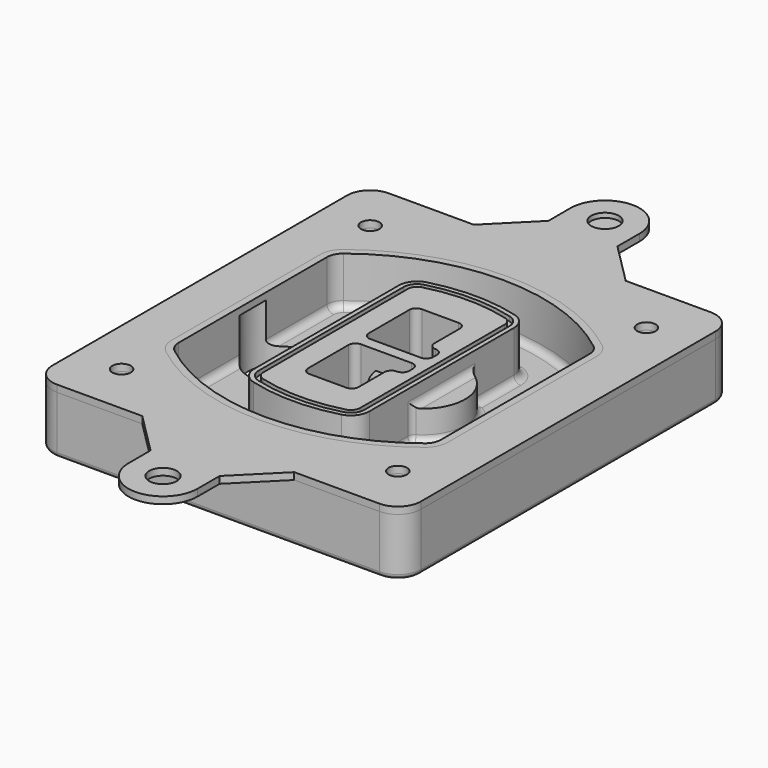
from build123d import *

# Parameters (mm, degrees)
F0_R      = 4
F1_DEPTH  = 25
F2_DEPTH  = 3
F3_DEPTH  = 18
F5_DEPTH  = 21
F6_DEPTH  = 2
F8_DEPTH  = 20
F9_DEPTH  = 16
F10_DEPTH = 25
F7_R      = 6
F7_R_2    = 4
F11_DEPTH = 6
F13_DEPTH = 9
F14_R     = 3
F15_R     = 2
F16_R     = 6
F16_R_2   = 4
F17_DEPTH = 3
F18_DEPTH = 1


# Not quite as in the source:
# - the program builds the solid bodies; features that only make, move or delete a surface that nothing else refers to are left out


with BuildPart() as f1:
    # F0 (on Top) → F1 (new body)
    with BuildSketch(Plane.XY):
        with BuildLine():
            ThreePointArc((-80, -80), (-77.0710678119, -87.0710678119), (-70, -90))
            Line((-70, -90), (70, -90))
            ThreePointArc((70, -90), (77.0710678119, -87.0710678119), (80, -80))
            Line((80, -80), (80, 80))
            ThreePointArc((80, 80), (77.0710678119, 87.0710678119), (70, 90))
            Line((70, 90), (-70, 90))
            ThreePointArc((-70, 90), (-77.0710678119, 87.0710678119), (-80, 80))
            Line((-80, 80), (-80, -80))
        make_face()
        with Locations((-60, -67.5)):
            Circle(F0_R, mode=Mode.SUBTRACT)
        with Locations((60, -67.5)):
            Circle(F0_R, mode=Mode.SUBTRACT)
        with Locations((-60, 67.5)):
            Circle(F0_R, mode=Mode.SUBTRACT)
        with BuildLine():
            ThreePointArc((-64, 40.2934422872), (-62.5820384798, 46.4328484224), (-58.6153846154, 51.3286200352))
            ThreePointArc((-58.6153846154, 51.3286200352), (0, 71.5), (58.6153846154, 51.3286200352))
            ThreePointArc((58.6153846154, 51.3286200352), (62.5820384798, 46.4328484224), (64, 40.2934422872))
            Line((64, 40.2934422872), (64, -40.2934422872))
            ThreePointArc((64, -40.2934422872), (62.5820384798, -46.4328484224), (58.6153846154, -51.3286200352))
            ThreePointArc((58.6153846154, -51.3286200352), (0, -71.5), (-58.6153846154, -51.3286200352))
            ThreePointArc((-58.6153846154, -51.3286200352), (-62.5820384798, -46.4328484224), (-64, -40.2934422872))
            Line((-64, -40.2934422872), (-64, 40.2934422872))
        make_face(mode=Mode.SUBTRACT)
        with Locations((60, 67.5)):
            Circle(F0_R, mode=Mode.SUBTRACT)
        with BuildLine():
            ThreePointArc((58.6153846154, 51.3286200352), (0, 71.5), (-58.6153846154, 51.3286200352))
            ThreePointArc((-58.6153846154, 51.3286200352), (-62.5820384798, 46.4328484224), (-64, 40.2934422872))
            Line((-64, 40.2934422872), (-64, -40.2934422872))
            ThreePointArc((-64, -40.2934422872), (-62.5820384798, -46.4328484224), (-58.6153846154, -51.3286200352))
            ThreePointArc((-58.6153846154, -51.3286200352), (0, -71.5), (58.6153846154, -51.3286200352))
            ThreePointArc((58.6153846154, -51.3286200352), (62.5820384798, -46.4328484224), (64, -40.2934422872))
            Line((64, -40.2934422872), (64, 40.2934422872))
            ThreePointArc((64, 40.2934422872), (62.5820384798, 46.4328484224), (58.6153846154, 51.3286200352))
        make_face()
        with BuildLine():
            Line((-60, -40.2934422872), (-60, 40.2934422872))
            ThreePointArc((-60, 40.2934422872), (-58.9871703427, 44.6787323838), (-56.1538461538, 48.1757121072))
            ThreePointArc((-56.1538461538, 48.1757121072), (0, 67.5), (56.1538461538, 48.1757121072))
            ThreePointArc((56.1538461538, 48.1757121072), (58.9871703427, 44.6787323838), (60, 40.2934422872))
            Line((60, 40.2934422872), (60, -40.2934422872))
            ThreePointArc((60, -40.2934422872), (58.9871703427, -44.6787323838), (56.1538461538, -48.1757121072))
            ThreePointArc((56.1538461538, -48.1757121072), (0, -67.5), (-56.1538461538, -48.1757121072))
            ThreePointArc((-56.1538461538, -48.1757121072), (-58.9871703427, -44.6787323838), (-60, -40.2934422872))
        make_face(mode=Mode.SUBTRACT)
        with BuildLine():
            ThreePointArc((-56.1538461538, 48.1757121072), (-58.9871703427, 44.6787323838), (-60, 40.2934422872))
            Line((-60, 40.2934422872), (-60, -40.2934422872))
            ThreePointArc((-60, -40.2934422872), (-58.9871703427, -44.6787323838), (-56.1538461538, -48.1757121072))
            ThreePointArc((-56.1538461538, -48.1757121072), (0, -67.5), (56.1538461538, -48.1757121072))
            ThreePointArc((56.1538461538, -48.1757121072), (58.9871703427, -44.6787323838), (60, -40.2934422872))
            Line((60, -40.2934422872), (60, 40.2934422872))
            ThreePointArc((60, 40.2934422872), (58.9871703427, 44.6787323838), (56.1538461538, 48.1757121072))
            ThreePointArc((56.1538461538, 48.1757121072), (0, 67.5), (-56.1538461538, 48.1757121072))
        make_face()
        with BuildLine():
            ThreePointArc((54.3076923077, 45.8110311612), (56.2910192399, 43.3631453548), (57, 40.2934422872))
            Line((57, 40.2934422872), (57, -40.2934422872))
            ThreePointArc((57, -40.2934422872), (56.2910192399, -43.3631453548), (54.3076923077, -45.8110311612))
            ThreePointArc((54.3076923077, -45.8110311612), (0, -64.5), (-54.3076923077, -45.8110311612))
            ThreePointArc((-54.3076923077, -45.8110311612), (-56.2910192399, -43.3631453548), (-57, -40.2934422872))
            Line((-57, -40.2934422872), (-57, 40.2934422872))
            ThreePointArc((-57, 40.2934422872), (-56.2910192399, 43.3631453548), (-54.3076923077, 45.8110311612))
            ThreePointArc((-54.3076923077, 45.8110311612), (0, 64.5), (54.3076923077, 45.8110311612))
        make_face(mode=Mode.SUBTRACT)
        with BuildLine():
            Line((57, -40.2934422872), (57, 40.2934422872))
            ThreePointArc((57, 40.2934422872), (56.2910192399, 43.3631453548), (54.3076923077, 45.8110311612))
            ThreePointArc((54.3076923077, 45.8110311612), (0, 64.5), (-54.3076923077, 45.8110311612))
            ThreePointArc((-54.3076923077, 45.8110311612), (-56.2910192399, 43.3631453548), (-57, 40.2934422872))
            Line((-57, 40.2934422872), (-57, -40.2934422872))
            ThreePointArc((-57, -40.2934422872), (-56.2910192399, -43.3631453548), (-54.3076923077, -45.8110311612))
            ThreePointArc((-54.3076923077, -45.8110311612), (0, -64.5), (54.3076923077, -45.8110311612))
            ThreePointArc((54.3076923077, -45.8110311612), (56.2910192399, -43.3631453548), (57, -40.2934422872))
        make_face()
    extrude(amount=-F1_DEPTH)

    # F0 (on Top) → F2 (join)
    with BuildSketch(Plane.XY):
        with BuildLine():
            ThreePointArc((-56.1538461538, 48.1757121072), (-58.9871703427, 44.6787323838), (-60, 40.2934422872))
            Line((-60, 40.2934422872), (-60, -40.2934422872))
            ThreePointArc((-60, -40.2934422872), (-58.9871703427, -44.6787323838), (-56.1538461538, -48.1757121072))
            ThreePointArc((-56.1538461538, -48.1757121072), (0, -67.5), (56.1538461538, -48.1757121072))
            ThreePointArc((56.1538461538, -48.1757121072), (58.9871703427, -44.6787323838), (60, -40.2934422872))
            Line((60, -40.2934422872), (60, 40.2934422872))
            ThreePointArc((60, 40.2934422872), (58.9871703427, 44.6787323838), (56.1538461538, 48.1757121072))
            ThreePointArc((56.1538461538, 48.1757121072), (0, 67.5), (-56.1538461538, 48.1757121072))
        make_face()
        with BuildLine():
            ThreePointArc((54.3076923077, 45.8110311612), (56.2910192399, 43.3631453548), (57, 40.2934422872))
            Line((57, 40.2934422872), (57, -40.2934422872))
            ThreePointArc((57, -40.2934422872), (56.2910192399, -43.3631453548), (54.3076923077, -45.8110311612))
            ThreePointArc((54.3076923077, -45.8110311612), (0, -64.5), (-54.3076923077, -45.8110311612))
            ThreePointArc((-54.3076923077, -45.8110311612), (-56.2910192399, -43.3631453548), (-57, -40.2934422872))
            Line((-57, -40.2934422872), (-57, 40.2934422872))
            ThreePointArc((-57, 40.2934422872), (-56.2910192399, 43.3631453548), (-54.3076923077, 45.8110311612))
            ThreePointArc((-54.3076923077, 45.8110311612), (0, 64.5), (54.3076923077, 45.8110311612))
        make_face(mode=Mode.SUBTRACT)
    extrude(amount=F2_DEPTH)

    # F0 (on Top) → F3 (cut)
    with BuildSketch(Plane.XY):
        with BuildLine():
            Line((57, -40.2934422872), (57, 40.2934422872))
            ThreePointArc((57, 40.2934422872), (56.2910192399, 43.3631453548), (54.3076923077, 45.8110311612))
            ThreePointArc((54.3076923077, 45.8110311612), (0, 64.5), (-54.3076923077, 45.8110311612))
            ThreePointArc((-54.3076923077, 45.8110311612), (-56.2910192399, 43.3631453548), (-57, 40.2934422872))
            Line((-57, 40.2934422872), (-57, -40.2934422872))
            ThreePointArc((-57, -40.2934422872), (-56.2910192399, -43.3631453548), (-54.3076923077, -45.8110311612))
            ThreePointArc((-54.3076923077, -45.8110311612), (0, -64.5), (54.3076923077, -45.8110311612))
            ThreePointArc((54.3076923077, -45.8110311612), (56.2910192399, -43.3631453548), (57, -40.2934422872))
        make_face()
    extrude(amount=-F3_DEPTH, mode=Mode.SUBTRACT)

    # F4 (on face) → F5 (join, through all)
    with BuildSketch(Plane.XY.offset(3)):
        with BuildLine():
            ThreePointArc((-25, -39.2465276821), (-23.3511545998, -44.1109737193), (-19.0842911877, -46.9702398883))
            ThreePointArc((-19.0842911877, -46.9702398883), (0, -49.5), (19.0842911877, -46.9702398883))
            ThreePointArc((19.0842911877, -46.9702398883), (23.3511545998, -44.1109737193), (25, -39.2465276821))
            Line((25, -39.2465276821), (25, 39.2465276821))
            ThreePointArc((25, 39.2465276821), (23.3511545998, 44.1109737193), (19.0842911877, 46.9702398883))
            ThreePointArc((19.0842911877, 46.9702398883), (0, 49.5), (-19.0842911877, 46.9702398883))
            ThreePointArc((-19.0842911877, 46.9702398883), (-23.3511545998, 44.1109737193), (-25, 39.2465276821))
            Line((-25, 39.2465276821), (-25, -39.2465276821))
        make_face()
        with BuildLine():
            ThreePointArc((18.5632183908, 45.0393118368), (21.7633659499, 42.89486221), (23, 39.2465276821))
            Line((23, 39.2465276821), (23, -39.2465276821))
            ThreePointArc((23, -39.2465276821), (21.7633659499, -42.89486221), (18.5632183908, -45.0393118368))
            ThreePointArc((18.5632183908, -45.0393118368), (0, -47.5), (-18.5632183908, -45.0393118368))
            ThreePointArc((-18.5632183908, -45.0393118368), (-21.7633659499, -42.89486221), (-23, -39.2465276821))
            Line((-23, -39.2465276821), (-23, 39.2465276821))
            ThreePointArc((-23, 39.2465276821), (-21.7633659499, 42.89486221), (-18.5632183908, 45.0393118368))
            ThreePointArc((-18.5632183908, 45.0393118368), (0, 47.5), (18.5632183908, 45.0393118368))
        make_face(mode=Mode.SUBTRACT)
        with BuildLine():
            Line((23, -39.2465276821), (23, 39.2465276821))
            ThreePointArc((23, 39.2465276821), (21.7633659499, 42.89486221), (18.5632183908, 45.0393118368))
            ThreePointArc((18.5632183908, 45.0393118368), (0, 47.5), (-18.5632183908, 45.0393118368))
            ThreePointArc((-18.5632183908, 45.0393118368), (-21.7633659499, 42.89486221), (-23, 39.2465276821))
            Line((-23, 39.2465276821), (-23, -39.2465276821))
            ThreePointArc((-23, -39.2465276821), (-21.7633659499, -42.89486221), (-18.5632183908, -45.0393118368))
            ThreePointArc((-18.5632183908, -45.0393118368), (0, -47.5), (18.5632183908, -45.0393118368))
            ThreePointArc((18.5632183908, -45.0393118368), (21.7633659499, -42.89486221), (23, -39.2465276821))
        make_face()
        with BuildLine():
            ThreePointArc((18.0421455939, 43.1083837852), (20.1755772999, 41.6787507007), (21, 39.2465276821))
            Line((21, 39.2465276821), (21, -39.2465276821))
            ThreePointArc((21, -39.2465276821), (20.1755772999, -41.6787507007), (18.0421455939, -43.1083837852))
            ThreePointArc((18.0421455939, -43.1083837852), (0, -45.5), (-18.0421455939, -43.1083837852))
            ThreePointArc((-18.0421455939, -43.1083837852), (-20.1755772999, -41.6787507007), (-21, -39.2465276821))
            Line((-21, -39.2465276821), (-21, 39.2465276821))
            ThreePointArc((-21, 39.2465276821), (-20.1755772999, 41.6787507007), (-18.0421455939, 43.1083837852))
            ThreePointArc((-18.0421455939, 43.1083837852), (0, 45.5), (18.0421455939, 43.1083837852))
        make_face(mode=Mode.SUBTRACT)
        with BuildLine():
            Line((21, -39.2465276821), (21, 39.2465276821))
            ThreePointArc((21, 39.2465276821), (20.1755772999, 41.6787507007), (18.0421455939, 43.1083837852))
            ThreePointArc((18.0421455939, 43.1083837852), (0, 45.5), (-18.0421455939, 43.1083837852))
            ThreePointArc((-18.0421455939, 43.1083837852), (-20.1755772999, 41.6787507007), (-21, 39.2465276821))
            Line((-21, 39.2465276821), (-21, -39.2465276821))
            ThreePointArc((-21, -39.2465276821), (-20.1755772999, -41.6787507007), (-18.0421455939, -43.1083837852))
            ThreePointArc((-18.0421455939, -43.1083837852), (0, -45.5), (18.0421455939, -43.1083837852))
            ThreePointArc((18.0421455939, -43.1083837852), (20.1755772999, -41.6787507007), (21, -39.2465276821))
        make_face()
        with BuildLine():
            Line((-8, -2.5), (14, -2.5))
            ThreePointArc((14, -2.5), (16.1213203436, -3.3786796564), (17, -5.5))
            Line((17, -5.5), (17, -7.5))
            ThreePointArc((17, -7.5), (16.1213203436, -9.6213203436), (14, -10.5))
            ThreePointArc((14, -10.5), (11.8786796564, -11.3786796564), (11, -13.5))
            Line((11, -13.5), (11, -27.5))
            ThreePointArc((11, -27.5), (10.1213203436, -29.6213203436), (8, -30.5))
            Line((8, -30.5), (-8, -30.5))
            ThreePointArc((-8, -30.5), (-10.1213203436, -29.6213203436), (-11, -27.5))
            Line((-11, -27.5), (-11, -5.5))
            ThreePointArc((-11, -5.5), (-10.1213203436, -3.3786796564), (-8, -2.5))
        make_face(mode=Mode.SUBTRACT)
        with BuildLine():
            ThreePointArc((-8, 2.5), (-10.1213203436, 3.3786796564), (-11, 5.5))
            Line((-11, 5.5), (-11, 27.5))
            ThreePointArc((-11, 27.5), (-10.1213203436, 29.6213203436), (-8, 30.5))
            Line((-8, 30.5), (8, 30.5))
            ThreePointArc((8, 30.5), (10.1213203436, 29.6213203436), (11, 27.5))
            Line((11, 27.5), (11, 13.5))
            ThreePointArc((11, 13.5), (11.8786796564, 11.3786796564), (14, 10.5))
            ThreePointArc((14, 10.5), (16.1213203436, 9.6213203436), (17, 7.5))
            Line((17, 7.5), (17, 5.5))
            ThreePointArc((17, 5.5), (16.1213203436, 3.3786796564), (14, 2.5))
            Line((14, 2.5), (-8, 2.5))
        make_face(mode=Mode.SUBTRACT)
    extrude(amount=-F5_DEPTH)

    # F4 (on face) → F6 (cut)
    with BuildSketch(Plane.XY.offset(3)):
        with BuildLine():
            Line((23, -39.2465276821), (23, 39.2465276821))
            ThreePointArc((23, 39.2465276821), (21.7633659499, 42.89486221), (18.5632183908, 45.0393118368))
            ThreePointArc((18.5632183908, 45.0393118368), (0, 47.5), (-18.5632183908, 45.0393118368))
            ThreePointArc((-18.5632183908, 45.0393118368), (-21.7633659499, 42.89486221), (-23, 39.2465276821))
            Line((-23, 39.2465276821), (-23, -39.2465276821))
            ThreePointArc((-23, -39.2465276821), (-21.7633659499, -42.89486221), (-18.5632183908, -45.0393118368))
            ThreePointArc((-18.5632183908, -45.0393118368), (0, -47.5), (18.5632183908, -45.0393118368))
            ThreePointArc((18.5632183908, -45.0393118368), (21.7633659499, -42.89486221), (23, -39.2465276821))
        make_face()
        with BuildLine():
            ThreePointArc((18.0421455939, 43.1083837852), (20.1755772999, 41.6787507007), (21, 39.2465276821))
            Line((21, 39.2465276821), (21, -39.2465276821))
            ThreePointArc((21, -39.2465276821), (20.1755772999, -41.6787507007), (18.0421455939, -43.1083837852))
            ThreePointArc((18.0421455939, -43.1083837852), (0, -45.5), (-18.0421455939, -43.1083837852))
            ThreePointArc((-18.0421455939, -43.1083837852), (-20.1755772999, -41.6787507007), (-21, -39.2465276821))
            Line((-21, -39.2465276821), (-21, 39.2465276821))
            ThreePointArc((-21, 39.2465276821), (-20.1755772999, 41.6787507007), (-18.0421455939, 43.1083837852))
            ThreePointArc((-18.0421455939, 43.1083837852), (0, 45.5), (18.0421455939, 43.1083837852))
        make_face(mode=Mode.SUBTRACT)
    extrude(amount=-F6_DEPTH, mode=Mode.SUBTRACT)

    # F7 (on face) → F8 (join)
    with BuildSketch(Plane(origin=(0, 0, -25), x_dir=(1, 0, 0), z_dir=(0, 0, -1))):
        with BuildLine():
            ThreePointArc((3.28842436, 0), (16.7567035675, 13.4682792075), (30.224982775, 0))
            Line((30.224982775, 0), (35.224982775, 0))
            ThreePointArc((35.224982775, 0), (16.7567035675, 18.4682792075), (-1.71157564, 0))
            Line((-1.71157564, 0), (3.28842436, 0))
        make_face()
        with BuildLine():
            Line((3.28842436, 0), (30.224982775, 0))
            ThreePointArc((30.224982775, 0), (16.7567035675, 13.4682792075), (3.28842436, 0))
        make_face()
        with BuildLine():
            ThreePointArc((3.28842436, 0), (16.7567035675, -13.4682792075), (30.224982775, 0))
            Line((30.224982775, 0), (3.28842436, 0))
        make_face()
        with BuildLine():
            Line((35.224982775, 0), (30.224982775, 0))
            ThreePointArc((30.224982775, 0), (16.7567035675, -13.4682792075), (3.28842436, 0))
            Line((3.28842436, 0), (-1.71157564, 0))
            ThreePointArc((-1.71157564, 0), (16.7567035675, -18.4682792075), (35.224982775, 0))
        make_face()
    extrude(amount=-F8_DEPTH)

    # F7 (on face) → F9 (cut)
    with BuildSketch(Plane(origin=(0, 0, -25), x_dir=(1, 0, 0), z_dir=(0, 0, -1))):
        with BuildLine():
            Line((3.28842436, 0), (30.224982775, 0))
            ThreePointArc((30.224982775, 0), (16.7567035675, 13.4682792075), (3.28842436, 0))
        make_face()
        with BuildLine():
            ThreePointArc((3.28842436, 0), (16.7567035675, -13.4682792075), (30.224982775, 0))
            Line((30.224982775, 0), (3.28842436, 0))
        make_face()
    extrude(amount=-F9_DEPTH, mode=Mode.SUBTRACT)

    # F7 (on face) → F10 (cut)
    with BuildSketch(Plane(origin=(0, 0, -25), x_dir=(1, 0, 0), z_dir=(0, 0, -1))):
        with BuildLine():
            Line((-59.0318229325, 0), (-32.0952645175, 0))
            ThreePointArc((-32.0952645175, 0), (-45.563543725, 13.4682792075), (-59.0318229325, 0))
        make_face()
        with BuildLine():
            ThreePointArc((-59.0318229325, 0), (-45.563543725, -13.4682792075), (-32.0952645175, 0))
            Line((-32.0952645175, 0), (-59.0318229325, 0))
        make_face()
    extrude(amount=-F10_DEPTH, mode=Mode.SUBTRACT)

    # F7 (on face) → F11 (cut)
    with BuildSketch(Plane(origin=(0, 0, -25), x_dir=(1, 0, 0), z_dir=(0, 0, -1))):
        with Locations((60, -67.5)):
            Circle(F7_R)
        with Locations((60, -67.5)):
            Circle(F7_R_2, mode=Mode.SUBTRACT)
        with Locations((-60, -67.5)):
            Circle(F7_R)
        with Locations((-60, -67.5)):
            Circle(F7_R_2, mode=Mode.SUBTRACT)
        with Locations((-60, 67.5)):
            Circle(F7_R)
        with Locations((-60, 67.5)):
            Circle(F7_R_2, mode=Mode.SUBTRACT)
        with Locations((60, 67.5)):
            Circle(F7_R)
        with Locations((60, 67.5)):
            Circle(F7_R_2, mode=Mode.SUBTRACT)
    extrude(amount=-F11_DEPTH, mode=Mode.SUBTRACT)

    # F12 (on face) → F13 (cut, through all)
    with BuildSketch(Plane(origin=(0, 0, -9), x_dir=(1, 0, 0), z_dir=(0, 0, -1))):
        with BuildLine():
            Line((11, 13.5), (11, 17.5481537753))
            ThreePointArc((11, 17.5481537753), (2.5696536419, 11.8239143813), (-1.5415842455, 2.5))
            Line((-1.5415842455, 2.5), (3.5224848595, 2.5))
            ThreePointArc((3.5224848595, 2.5), (6.1857188154, 8.3455872281), (11.2536447004, 12.2927168648))
            ThreePointArc((11.2536447004, 12.2927168648), (11.0640958889, 12.8831798879), (11, 13.5))
        make_face()
        with BuildLine():
            ThreePointArc((11.2536447004, -12.2927168648), (6.1857188154, -8.3455872281), (3.5224848595, -2.5))
            Line((3.5224848595, -2.5), (-1.5415842455, -2.5))
            ThreePointArc((-1.5415842455, -2.5), (2.5696536419, -11.8239143813), (11, -17.5481537753))
            Line((11, -17.5481537753), (11, -13.5))
            ThreePointArc((11, -13.5), (11.0640958889, -12.8831798879), (11.2536447004, -12.2927168648))
        make_face()
        with BuildLine():
            ThreePointArc((11.2536447004, 12.2927168648), (6.1857188154, 8.3455872281), (3.5224848595, 2.5))
            Line((3.5224848595, 2.5), (14, 2.5))
            ThreePointArc((14, 2.5), (16.1213203436, 3.3786796564), (17, 5.5))
            Line((17, 5.5), (17, 7.5))
            ThreePointArc((17, 7.5), (16.1213203436, 9.6213203436), (14, 10.5))
            ThreePointArc((14, 10.5), (12.3601599782, 10.9878446101), (11.2536447004, 12.2927168648))
        make_face()
        with BuildLine():
            Line((14, -2.5), (3.5224848595, -2.5))
            ThreePointArc((3.5224848595, -2.5), (6.1857188154, -8.3455872281), (11.2536447004, -12.2927168648))
            ThreePointArc((11.2536447004, -12.2927168648), (12.3601599782, -10.9878446101), (14, -10.5))
            ThreePointArc((14, -10.5), (16.1213203436, -9.6213203436), (17, -7.5))
            Line((17, -7.5), (17, -5.5))
            ThreePointArc((17, -5.5), (16.1213203436, -3.3786796564), (14, -2.5))
        make_face()
    extrude(amount=F13_DEPTH, mode=Mode.SUBTRACT)

    # F14
    f14_edges = [f1.edges().sort_by_distance(p)[0] for p in [
        (-57, -23.703476, -18),
        (-57, 23.703476, -18),
        (25, 0, -5),
        (25, 16.526506, -11.5),
        (25, -16.526506, -11.5),
        (25, -27.886517, -18),
        (35.224983, 0, -18),
    ]]
    fillet(f14_edges, radius=F14_R)

    # F15
    f15_edges = [f1.edges().sort_by_distance(p)[0] for p in [
        (0, -90, -25),
    ]]
    fillet(f15_edges, radius=F15_R)


with BuildPart() as f17:
    # F16 (on face) → F17 (new body, through all)
    with BuildSketch(Plane.XY):
        with BuildLine():
            Line((-15, 108), (-33, 90))
            Line((-33, 90), (33, 90))
            Line((33, 90), (15, 108))
            Line((15, 108), (15, 120))
            ThreePointArc((15, 120), (0, 135), (-15, 120))
            Line((-15, 120), (-15, 108))
        make_face()
        with Locations((0, 120)):
            Circle(F16_R, mode=Mode.SUBTRACT)
        with BuildLine():
            Line((33, -90), (-33, -90))
            Line((-33, -90), (-15, -108))
            Line((-15, -108), (-15, -120))
            ThreePointArc((-15, -120), (0, -135), (15, -120))
            Line((15, -120), (15, -108))
            Line((15, -108), (33, -90))
        make_face()
        with Locations((0, -120)):
            Circle(F16_R, mode=Mode.SUBTRACT)
        with BuildLine():
            Line((-33, 90), (-70, 90))
            ThreePointArc((-70, 90), (-77.0710678119, 87.0710678119), (-80, 80))
            Line((-80, 80), (-80, -80))
            ThreePointArc((-80, -80), (-77.0710678119, -87.0710678119), (-70, -90))
            Line((-70, -90), (-33, -90))
            Line((-33, -90), (33, -90))
            Line((33, -90), (70, -90))
            ThreePointArc((70, -90), (77.0710678119, -87.0710678119), (80, -80))
            Line((80, -80), (80, 80))
            ThreePointArc((80, 80), (77.0710678119, 87.0710678119), (70, 90))
            Line((70, 90), (33, 90))
            Line((33, 90), (-33, 90))
        make_face()
        with Locations((-60, -67.5)):
            Circle(F16_R_2, mode=Mode.SUBTRACT)
        with Locations((60, -67.5)):
            Circle(F16_R_2, mode=Mode.SUBTRACT)
        with Locations((-60, 67.5)):
            Circle(F16_R_2, mode=Mode.SUBTRACT)
        with BuildLine():
            ThreePointArc((56.1538461538, -48.1757121072), (0, -67.5), (-56.1538461538, -48.1757121072))
            ThreePointArc((-56.1538461538, -48.1757121072), (-58.9871703427, -44.6787323838), (-60, -40.2934422872))
            Line((-60, -40.2934422872), (-60, 40.2934422872))
            ThreePointArc((-60, 40.2934422872), (-58.9871703427, 44.6787323838), (-56.1538461538, 48.1757121072))
            ThreePointArc((-56.1538461538, 48.1757121072), (0, 67.5), (56.1538461538, 48.1757121072))
            ThreePointArc((56.1538461538, 48.1757121072), (58.9871703427, 44.6787323838), (60, 40.2934422872))
            Line((60, 40.2934422872), (60, -40.2934422872))
            ThreePointArc((60, -40.2934422872), (58.9871703427, -44.6787323838), (56.1538461538, -48.1757121072))
        make_face(mode=Mode.SUBTRACT)
        with Locations((60, 67.5)):
            Circle(F16_R_2, mode=Mode.SUBTRACT)
    extrude(amount=F17_DEPTH)

    # F16 (on face) → F18 (join, through all)
    with BuildSketch(Plane.XY):
        with Locations((0, 120)):
            Circle(F16_R)
    extrude(amount=F18_DEPTH)


solid = Compound([f1.part, f17.part])
